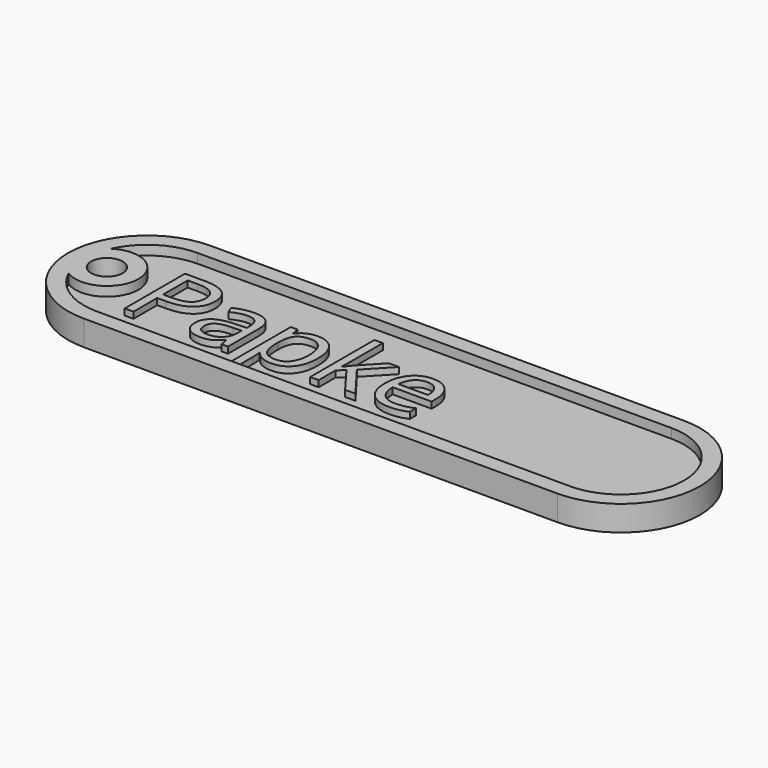
from build123d import *

# Parameters (mm, degrees)
F1_DEPTH     = 101.6
F3_DEPTH     = 38.1
F4_R         = 63.5
F5_DEPTH     = 101.6
F6_TEXT_SIZE = 424.1197722628
F7_DEPTH     = 25.4


# Not quite as in the source:
# - Text() gives the source's letters only with a copy of the font that has no kerning and outlines rounded to 1/6400 em; it was checked with that copy


with BuildPart() as f1:
    # F0 (on Top) → F1 (new body)
    with BuildSketch(Plane.XY):
        with BuildLine():
            ThreePointArc((0, 635), (-317.5, 317.5), (0, 0))
            Line((0, 0), (1905, 0))
            ThreePointArc((1905, 0), (2222.5, 317.5), (1905, 635))
            Line((1905, 635), (0, 635))
        make_face()
    extrude(amount=F1_DEPTH)

    # F2 (on face) → F3 (cut)
    with BuildSketch(Plane.XY.offset(101.6)):
        with BuildLine():
            Line((1905, 571.5), (0, 571.5))
            ThreePointArc((0, 571.5), (-136.8621840783, 531.4736959752), (-230.5898217834, 424.0097840103))
            ThreePointArc((-230.5898217834, 424.0097840103), (-34.4185422659, 317.5), (-230.5898217834, 210.9902159897))
            ThreePointArc((-230.5898217834, 210.9902159897), (-136.8621840783, 103.5263040248), (0, 63.5))
            Line((0, 63.5), (1905, 63.5))
            ThreePointArc((1905, 63.5), (2159, 317.5), (1905, 571.5))
        make_face()
    extrude(amount=-F3_DEPTH, mode=Mode.SUBTRACT)

    # F4 (on face) → F5 (cut)
    with BuildSketch(Plane.XY.offset(101.6)):
        with Locations((-161.4185422659, 317.5)):
            Circle(F4_R)
    extrude(amount=-F5_DEPTH, mode=Mode.SUBTRACT)

    # F6 (on face) → F7 (join)
    with BuildSketch(Plane.XY.offset(63.5)):
        with Locations((0, 153.0302909481)):
            Text('Papke', F6_TEXT_SIZE, font='Open Sans', text_align=(TextAlign.LEFT, TextAlign.BOTTOM))
    extrude(amount=F7_DEPTH)


solid = f1.part
